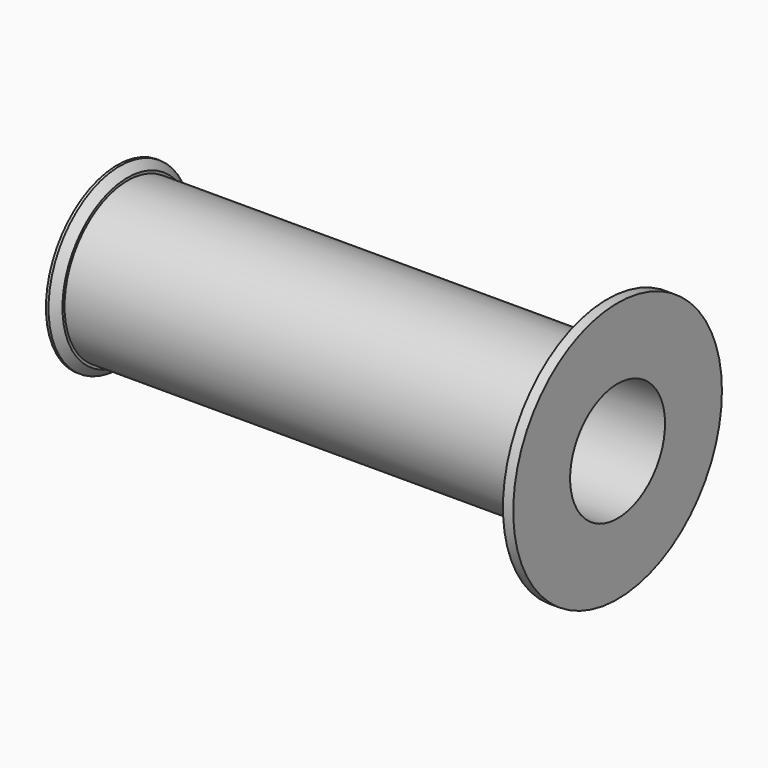
from build123d import *

# Parameters (mm, degrees)
F2_SIZE  = 1.5
F3_R     = 7
F4_DEPTH = 75.001


# Not quite as in the source:
# - a feature names something its author has since deleted; it is built from what else it names


with BuildPart() as f1:
    # F0 (on Top) → F1 (revolve)
    with BuildSketch(Plane.XY):
        with BuildLine():
            Line((-18.3783795104, 0), (31.6216204896, 0))
            Line((31.6216204896, 0), (31.6216204896, 11.5))
            Line((31.6216204896, 11.5), (53.6216204896, 11.5))
            Line((53.6216204896, 11.5), (53.6216204896, 15.2837846328))
            Line((53.6216204896, 15.2837846328), (53.6216204896, 25.2837846328))
            Line((53.6216204896, 25.2837846328), (51.6216204896, 25.2837846328))
            Line((51.6216204896, 25.2837846328), (51.6216204896, 15.2837846328))
            Line((51.6216204896, 15.2837846328), (39.6216204896, 15.2837846328))
            Line((39.6216204896, 15.2837846328), (-41.3783795104, 15.2837846328))
            Line((-41.3783795104, 15.2837846328), (-41.3783795104, 17.2837846328))
            Line((-41.3783795104, 17.2837846328), (-43.3783795104, 17.2837846328))
            Line((-43.3783795104, 17.2837846328), (-43.3783795104, 15.2837846328))
            Line((-43.3783795104, 15.2837846328), (-43.3783795104, 11.5))
            Line((-43.3783795104, 11.5), (-28.3783795104, 11.5))
            ThreePointArc((-28.3783795104, 11.5), (-21.3073116985, 8.5710678119), (-18.3783795104, 1.5))
            Line((-18.3783795104, 1.5), (-18.3783795104, 0))
        make_face()
    revolve(axis=Axis((6.6216204896, 0, 0), (-1, 0, 0)))

    # F2
    f2_edges = [f1.edges().sort_by_distance(p)[0] for p in [
        (-41.37838, -17.283785, 0),
    ]]
    chamfer(f2_edges, length=F2_SIZE)

    # F3 (on face) → F4 (cut, through all)
    with BuildSketch(Plane.YZ.offset(31.6216204896)):
        Circle(F3_R)
    extrude(amount=-F4_DEPTH, mode=Mode.SUBTRACT)


solid = f1.part
